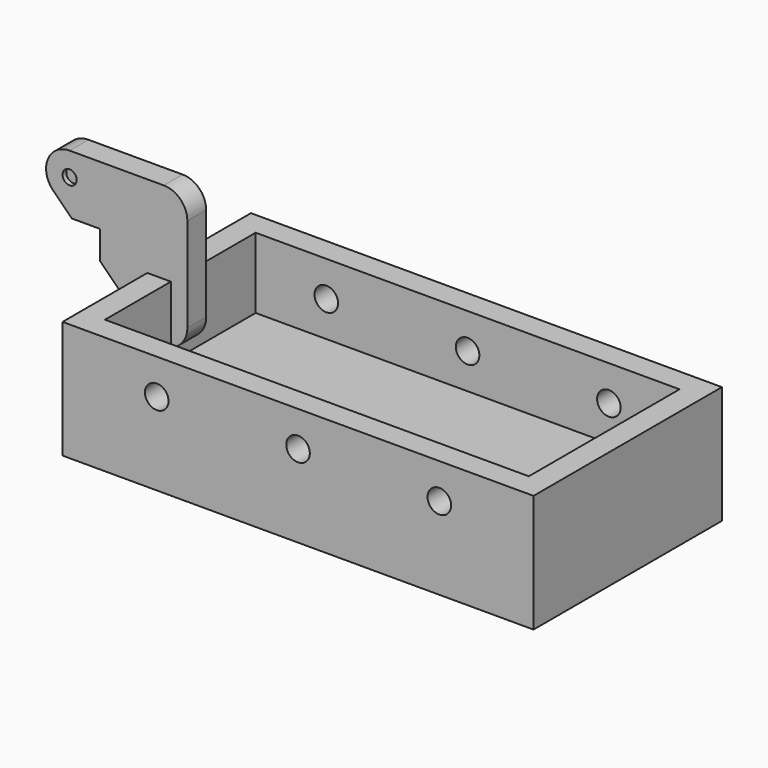
from build123d import *

# Parameters (mm, degrees)
F0_W      = 100
F0_H      = 50
F0_W_2    = 90
F0_H_2    = 40
F1_DEPTH  = 7.5
F2_R      = 2.5
F3_DEPTH  = 50.001
F4_W      = 100
F4_H      = 50
F4_W_2    = 90
F4_H_2    = 40
F5_DEPTH  = 10
F7_DEPTH  = 2.5
F8_R      = 1.5
F9_DEPTH  = 1
F10_R     = 1.5
F11_DEPTH = 1
F13_DEPTH = 27.501


with BuildPart() as f1:
    # F0 (on Top) → F1 (new body, symmetric)
    with BuildSketch(Plane.XY):
        Rectangle(F0_W, F0_H)
        Rectangle(F0_W_2, F0_H_2, mode=Mode.SUBTRACT)
    extrude(amount=F1_DEPTH, both=True)

    # F2 (on face) → F3 (cut, through all)
    with BuildSketch(Plane.XZ.offset(25)):
        Circle(F2_R)
        with Locations((-30, 0)):
            Circle(F2_R)
        with Locations((30, 0)):
            Circle(F2_R)
    extrude(amount=-F3_DEPTH, mode=Mode.SUBTRACT)

    # F4 (on face) → F5 (join)
    with BuildSketch(Plane(origin=(0, 0, -7.5), x_dir=(1, 0, 0), z_dir=(0, 0, -1))):
        Rectangle(F4_W, F4_H)
        Rectangle(F4_W_2, F4_H_2, mode=Mode.SUBTRACT)
        Rectangle(F4_W_2, F4_H_2)
    extrude(amount=F5_DEPTH)

    # F6 (on Front) → F7 (join, symmetric)
    with BuildSketch(Plane.XZ):
        with BuildLine():
            Line((-70.0356467673, 16.4644660941), (-50.0356467673, -3.5355339059))
            ThreePointArc((-50.0356467673, -3.5355339059), (-44.5866956996, -4.6193976626), (-41.5001128614, 0))
            Line((-41.5001128614, 0), (-41.5001128614, 20))
            ThreePointArc((-41.5001128614, 20), (-42.9645789555, 23.5355339059), (-46.5001128614, 25))
            Line((-46.5001128614, 25), (-66.5001128614, 25))
            ThreePointArc((-66.5001128614, 25), (-71.119510524, 21.9134171618), (-70.0356467673, 16.4644660941))
        make_face()
    extrude(amount=F7_DEPTH, both=True)

    # F8 (on face) → F9 (cut)
    with BuildSketch(Plane.XZ.offset(2.5)):
        with Locations((-66.5001128614, 20)):
            Circle(F8_R)
    extrude(amount=-F9_DEPTH, mode=Mode.SUBTRACT)

    # F10 (on face) → F11 (cut)
    with BuildSketch(Plane(origin=(0, 2.5, 0), x_dir=(-1, 0, 0), z_dir=(0, 1, 0))):
        with Locations((66.5001128614, 20)):
            Circle(F10_R)
    extrude(amount=-F11_DEPTH, mode=Mode.SUBTRACT)

    # F12 (on face) → F13 (cut, through all)
    with BuildSketch(Plane.XZ.offset(2.5)):
        Polygon((-60.0356467673, 12.4644660941), (-66.0356467673, 12.4644660941), (-60.0356467673, 6.4644660941), align=None)
    extrude(amount=-F13_DEPTH, mode=Mode.SUBTRACT)


solid = f1.part
